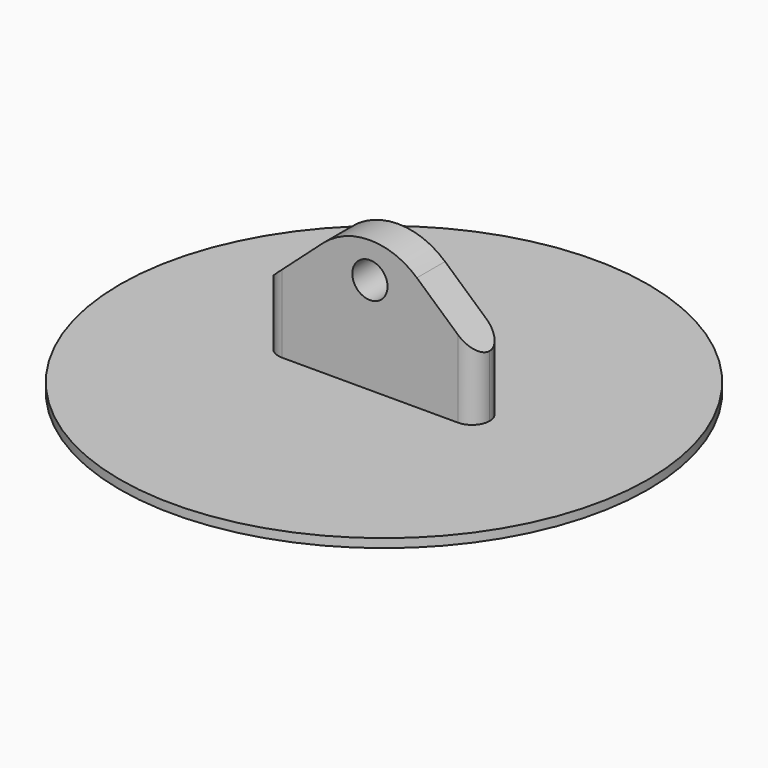
from build123d import *

# Parameters (mm, degrees)
F0_R     = 95.25
F1_DEPTH = 3.175
F3_DEPTH = 6.35
F4_R     = 6.34999


# Not quite as in the source:
# - a fillet or chamfer is up to 0.001 mm smaller than in the source, because OpenCascade refuses the exact size


with BuildPart() as f1:
    # F0 (on Top) → F1 (new body)
    with BuildSketch(Plane.XY):
        Circle(F0_R)
    extrude(amount=F1_DEPTH)

    # F2 (on Front) → F3 (join, symmetric)
    with BuildSketch(Plane.XZ):
        with BuildLine():
            Line((38.1, 0), (38.1, 25.4))
            Line((38.1, 25.4), (16.9333333333, 44.3320422095))
            ThreePointArc((16.9333333333, 44.3320422095), (0, 50.8), (-16.9333333333, 44.3320422095))
            Line((-16.9333333333, 44.3320422095), (-38.1, 25.4))
            Line((-38.1, 25.4), (-38.1, 0))
            Line((-38.1, 0), (0, 0))
            Line((0, 0), (38.1, 0))
        make_face()
        with BuildLine():
            ThreePointArc((6.35, 38.1), (4.4901280605, 33.6098719395), (0, 31.75))
            ThreePointArc((0, 31.75), (-4.4901280605, 42.5901280605), (6.35, 38.1))
        make_face(mode=Mode.SUBTRACT)
    extrude(amount=F3_DEPTH, both=True)

    # F4 (radius 6.35 in the source; OpenCascade refuses exactly that, so slightly less here)
    f4_edges = [f1.edges().sort_by_distance(p)[0] for p in [
        (-38.1, -6.35, 14.2875),
        (-38.1, 6.35, 14.2875),
        (38.1, -6.35, 14.2875),
        (38.1, 6.35, 14.2875),
    ]]
    fillet(f4_edges, radius=F4_R)


solid = f1.part
